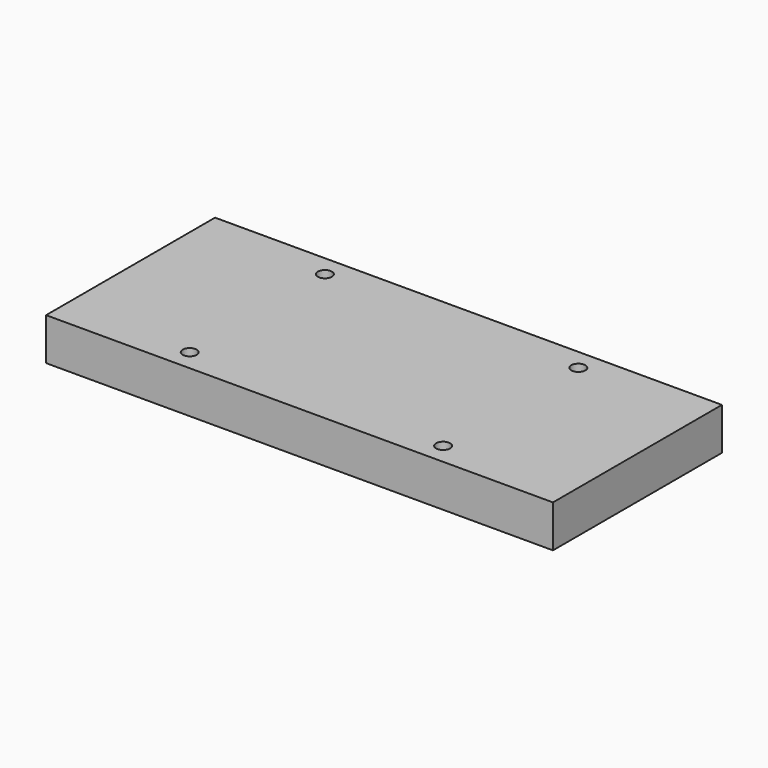
from build123d import *

# Parameters (mm, degrees)
F0_W       = 457.2
F0_H       = 38.1
F1_DEPTH   = 95.25
F4_D       = 12.7
F4_DEPTH   = 609.6
F4_TIP     = 3.8154649308
F4_2_D     = 12.7
F4_2_DEPTH = 609.6
F4_2_TIP   = 3.8154649308
F5_D       = 12.7
F5_DEPTH   = 609.6
F5_TIP     = 3.8154649308
F5_2_D     = 12.7
F5_2_DEPTH = 609.6
F5_2_TIP   = 3.8154649308
F6_D       = 12.7
F6_DEPTH   = 609.6
F6_TIP     = 3.8154649308
F6_2_D     = 12.7
F6_2_DEPTH = 609.6
F6_2_TIP   = 3.8154649308
F7_D       = 12.7
F7_DEPTH   = 609.6
F7_TIP     = 3.8154649308
F7_2_D     = 12.7
F7_2_DEPTH = 609.6
F7_2_TIP   = 3.8154649308


# Not quite as in the source:
# - a feature names something its author has since deleted; it is built from what else it names


with BuildPart() as f1:
    # F0 (on Front) → F1 (new body, symmetric)
    with BuildSketch(Plane.XZ):
        Rectangle(F0_W, F0_H)
    extrude(amount=F1_DEPTH, both=True)


with BuildPart() as f2_1:
    # F2: copy of F1
    add(f1.part.moved(Location((0, 0, 152.4))))

    # F4#2
    with Locations(Plane.XY.offset(171.45)):
        with Locations((-114.3, 76.2)):
            Hole(F4_2_D / 2, depth=F4_2_DEPTH)
            with Locations((0, 0, -(F4_2_DEPTH + F4_2_TIP / 2))):  # 118° drill point
                Cone(0, F4_2_D / 2, F4_2_TIP, mode=Mode.SUBTRACT)

    # F5#2
    with Locations(Plane.XY.offset(171.45)):
        with Locations((114.3, 76.2)):
            Hole(F5_2_D / 2, depth=F5_2_DEPTH)
            with Locations((0, 0, -(F5_2_DEPTH + F5_2_TIP / 2))):  # 118° drill point
                Cone(0, F5_2_D / 2, F5_2_TIP, mode=Mode.SUBTRACT)

    # F6#2
    with Locations(Plane.XY.offset(171.45)):
        with Locations((-114.3, -76.2)):
            Hole(F6_2_D / 2, depth=F6_2_DEPTH)
            with Locations((0, 0, -(F6_2_DEPTH + F6_2_TIP / 2))):  # 118° drill point
                Cone(0, F6_2_D / 2, F6_2_TIP, mode=Mode.SUBTRACT)

    # F7#2
    with Locations(Plane.XY.offset(171.45)):
        with Locations((114.3, -76.2)):
            Hole(F7_2_D / 2, depth=F7_2_DEPTH)
            with Locations((0, 0, -(F7_2_DEPTH + F7_2_TIP / 2))):  # 118° drill point
                Cone(0, F7_2_D / 2, F7_2_TIP, mode=Mode.SUBTRACT)


with BuildPart() as f1_1:
    add(f1.part)

    # F4
    with Locations(Plane.XY.offset(171.45)):
        with Locations((-114.3, 76.2)):
            Hole(F4_D / 2, depth=F4_DEPTH)
            with Locations((0, 0, -(F4_DEPTH + F4_TIP / 2))):  # 118° drill point
                Cone(0, F4_D / 2, F4_TIP, mode=Mode.SUBTRACT)

    # F5
    with Locations(Plane.XY.offset(171.45)):
        with Locations((114.3, 76.2)):
            Hole(F5_D / 2, depth=F5_DEPTH)
            with Locations((0, 0, -(F5_DEPTH + F5_TIP / 2))):  # 118° drill point
                Cone(0, F5_D / 2, F5_TIP, mode=Mode.SUBTRACT)

    # F6
    with Locations(Plane.XY.offset(171.45)):
        with Locations((-114.3, -76.2)):
            Hole(F6_D / 2, depth=F6_DEPTH)
            with Locations((0, 0, -(F6_DEPTH + F6_TIP / 2))):  # 118° drill point
                Cone(0, F6_D / 2, F6_TIP, mode=Mode.SUBTRACT)

    # F7
    with Locations(Plane.XY.offset(171.45)):
        with Locations((114.3, -76.2)):
            Hole(F7_D / 2, depth=F7_DEPTH)
            with Locations((0, 0, -(F7_DEPTH + F7_TIP / 2))):  # 118° drill point
                Cone(0, F7_D / 2, F7_TIP, mode=Mode.SUBTRACT)


solid = f1_1.part
